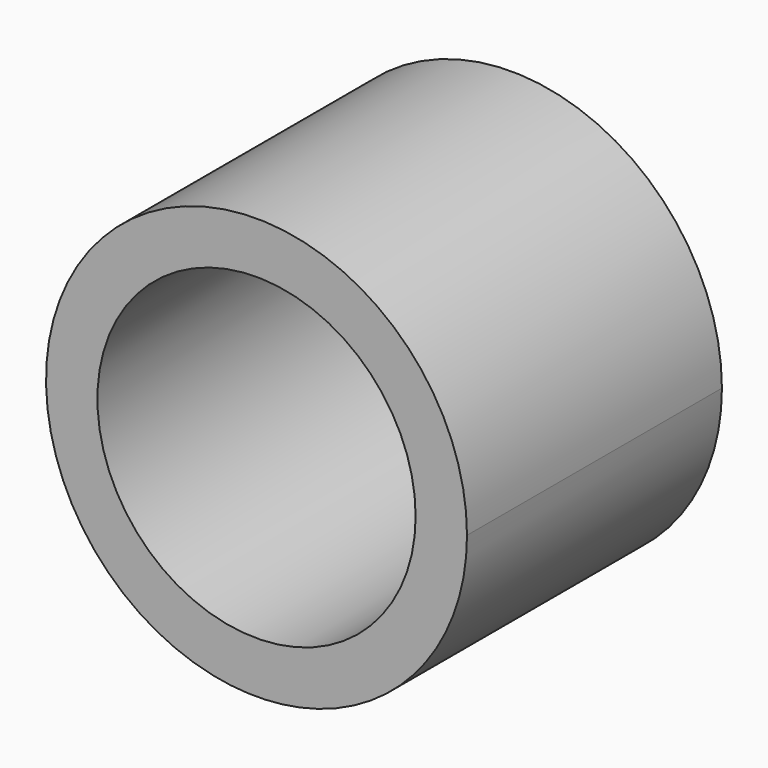
from build123d import *

# Parameters (mm, degrees)
F1_DEPTH = 25
F2_R     = 12.4828054131
F3_DEPTH = 30
F5_R     = 1.2870142299
F6_DEPTH = 1.5


with BuildPart() as f1:
    # F0 (on Front) → F1 (new body)
    with BuildSketch(Plane.XZ):
        with BuildLine():
            Line((-3.388106823, -14.5254029512), (-3.388106823, -16.1620440826))
            ThreePointArc((-3.388106823, -16.1620440826), (0, -16.5133563146), (3.388106823, -16.1620440826))
            Line((3.388106823, -16.1620440826), (3.388106823, -14.5254029512))
            Line((3.388106823, -14.5254029512), (-3.388106823, -14.5254029512))
        make_face()
        with BuildLine():
            ThreePointArc((3.388106823, -16.1620440826), (12.8187353505, -10.4101374048), (16.5133563146, 0))
            ThreePointArc((16.5133563146, 0), (-10.4101374048, 12.8187353505), (-3.388106823, -16.1620440826))
            Line((-3.388106823, -16.1620440826), (-3.388106823, -14.5254029512))
            Line((-3.388106823, -14.5254029512), (3.388106823, -14.5254029512))
            Line((3.388106823, -14.5254029512), (3.388106823, -16.1620440826))
        make_face()
    extrude(amount=F1_DEPTH)

    # F2 (on face) → F3 (cut)
    with BuildSketch(Plane.XZ.offset(25)):
        Circle(F2_R)
    extrude(amount=-F3_DEPTH, mode=Mode.SUBTRACT)


with BuildPart() as f6:
    # F5 (on face) → F6 (new body, symmetric)
    with BuildSketch(Plane.XY.offset(-18.501309678)):
        with Locations((0, -12.5)):
            Circle(F5_R)
    extrude(amount=F6_DEPTH, both=True)


solid = Compound([f1.part, f6.part])
